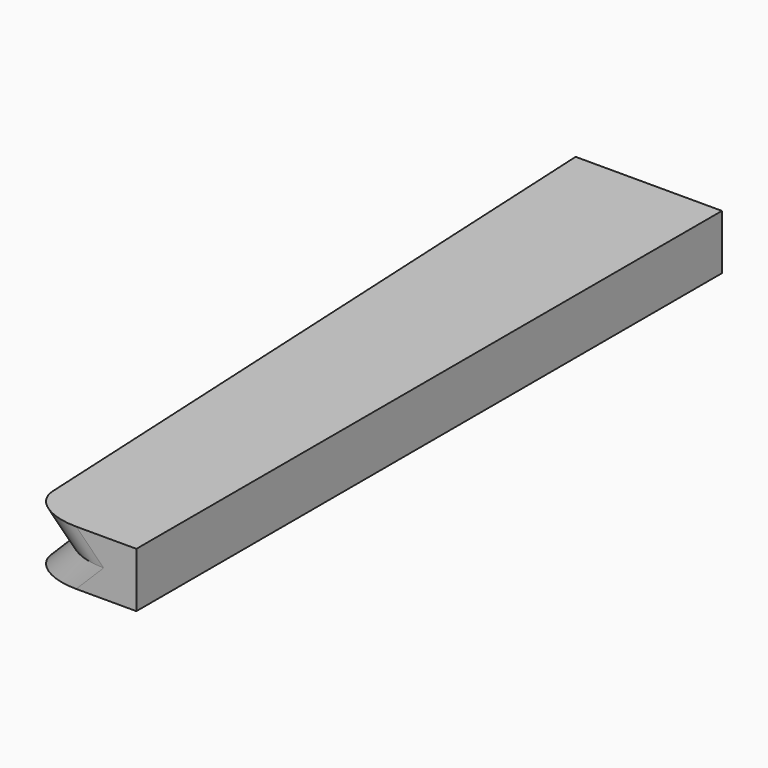
from build123d import *

# Parameters (mm, degrees)
F1_DEPTH     = 200
F2_T1_DEPTH  = 531.7746698901
F2_T3_DEPTH  = 531.7746698901
F2_T9_DEPTH  = 1052.9427380625
F2_T14_DEPTH = 1052.9427380625
F3_R         = 10


# Not quite as in the source:
# - a fillet or chamfer that OpenCascade refuses, or shapes differently, is made with other operations: its cross-section is extruded or revolved along the edge and cut away or added


with BuildPart() as f1:
    # F0 (on Front) → F1 (new body)
    with BuildSketch(Plane.XZ):
        Polygon((-25, 0), (0, 0), (0, 15), (-40, 15), (-32.5, 7.5), (-40, 0), align=None)
    extrude(amount=F1_DEPTH)

    # F2: chamfer of 7 x 200.4537729804 on 2 edges, made by hand

    # F2_s2 → F2_t1 (cut)
    with BuildSketch(Plane(origin=(-396.0214751426, 0, 396.0214751426), x_dir=(0, 1, 0), z_dir=(0.7071067812, 0, -0.7071067812))):
        Polygon((-200, -10.6776695297), (0.4537729804, -17.6776695297), (-200, -17.6776695297), align=None)
    extrude(amount=F2_T1_DEPTH, mode=Mode.SUBTRACT)

    # F2_s4 → F2_t3 (cut)
    with BuildSketch(Plane(origin=(-12.5, 0, -12.5), x_dir=(0, 1, 0), z_dir=(-0.7071067812, 0, -0.7071067812))):
        Polygon((-200, -21.2842712475), (0.4537729804, -28.2842712475), (-200, -28.2842712475), align=None)
    extrude(amount=F2_T3_DEPTH, mode=Mode.SUBTRACT)


with BuildPart() as f2_tool7:
    # F2_s8 → F2_t9 (new body)
    with BuildSketch(Plane(origin=(-396.0214751426, 0, 396.0214751426), x_dir=(0, 1, 0), z_dir=(0.7071067812, 0, -0.7071067812))):
        Polygon((-200, -10.6776695297), (0.4537729804, -17.6776695297), (-200, -17.6776695297), align=None)
    extrude(amount=F2_T9_DEPTH)

    split(bisect_by=Plane.XY, keep=Keep.TOP)

    split(bisect_by=Plane(origin=(-20, 0, 20), x_dir=(0, 1, 0), z_dir=(0.7071067812, 0, -0.7071067812)), keep=Keep.TOP)


with BuildPart() as f2_tool12:
    # F2_s13 → F2_t14 (new body)
    with BuildSketch(Plane(origin=(356.0214751426, 0, 356.0214751426), x_dir=(0, 1, 0), z_dir=(-0.7071067812, 0, -0.7071067812))):
        Polygon((-200, -21.2842712475), (0.4537729804, -28.2842712475), (-200, -28.2842712475), align=None)
    extrude(amount=F2_T14_DEPTH)

    split(bisect_by=Plane(origin=(-12.5, 0, -12.5), x_dir=(0, 1, 0), z_dir=(0.7071067812, 0, 0.7071067812)), keep=Keep.TOP)

    split(bisect_by=Plane.XY.offset(15), keep=Keep.BOTTOM)


with BuildPart() as f2_tool7_1:
    add(f2_tool7.part)

    # F2_t17: intersect F2_tool12
    add(f2_tool12.part, mode=Mode.INTERSECT)


with BuildPart() as f1_1:
    add(f1.part)

    # F2_t5: cut F2_tool7
    add(f2_tool7_1.part, mode=Mode.SUBTRACT)

    # F3
    f3_edges = [f1_1.edges().sort_by_distance(p)[0] for p in [
        (-26.350505, -200, 11.25),
        (-26.350505, -200, 3.75),
    ]]
    fillet(f3_edges, radius=F3_R)


solid = f1_1.part
